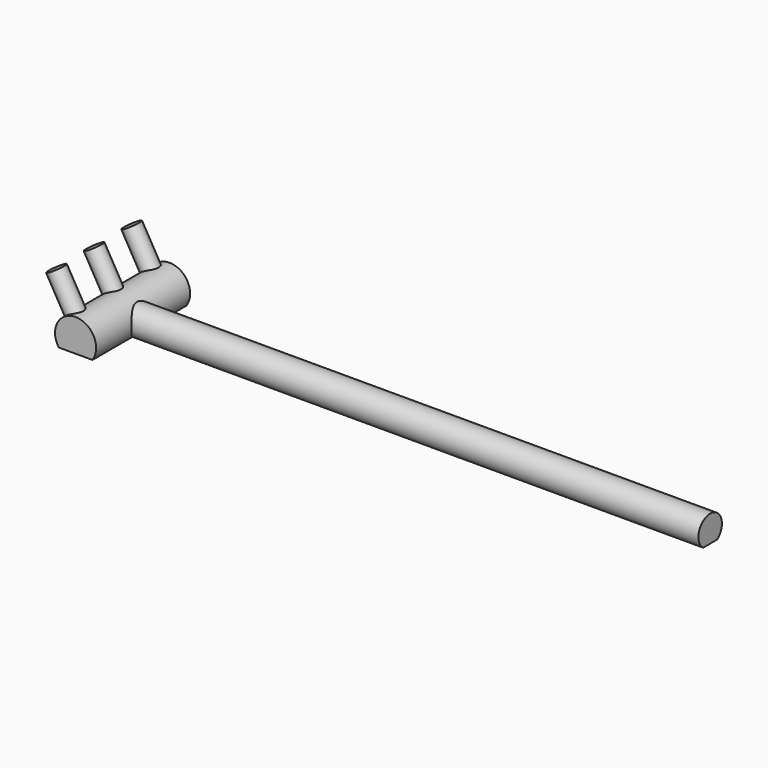
from build123d import *

# Parameters (mm, degrees)
F1_DEPTH        = 10
F3_DEPTH        = 100
F5_R            = 1.5
F6_DEPTH        = 10
F6_COPIES_COUNT = 2
F6_COPIES_PITCH = 8


# Not quite as in the source:
# - a pattern or mirror of a feature is missing from the dataset's text; its kind, count and spacing are read off the source's solid


with BuildPart() as f1:
    # F0 (on Front) → F1 (new body, symmetric)
    with BuildSketch(Plane.XZ):
        with BuildLine():
            Line((-2.8722813233, -2), (2.8722813233, -2))
            ThreePointArc((2.8722813233, -2), (0, 3.5), (-2.8722813233, -2))
        make_face()
    extrude(amount=F1_DEPTH, both=True)

    # F2 (on Right) → F3 (join)
    with BuildSketch(Plane.YZ):
        with BuildLine():
            Line((-1.5, -2), (1.5, -2))
            ThreePointArc((1.5, -2), (0, 2.5), (-1.5, -2))
        make_face()
    extrude(amount=F3_DEPTH)

    # F5 (on face) → F6 (join)
    with BuildSketch(Plane(origin=(0.147955073, 0, -0.2562657036), x_dir=(0.8660254038, 0, 0.5), z_dir=(0.5, 0, -0.8660254038))):
        Circle(F5_R)
        with Locations((0, -8)):
            Circle(F5_R)
    f6 = extrude(amount=-F6_DEPTH)

    # F6_copies: F6 ×2
    with Locations(*[(0, -i * F6_COPIES_PITCH, 0) for i in range(1, F6_COPIES_COUNT)]):
        add(f6)


solid = f1.part
